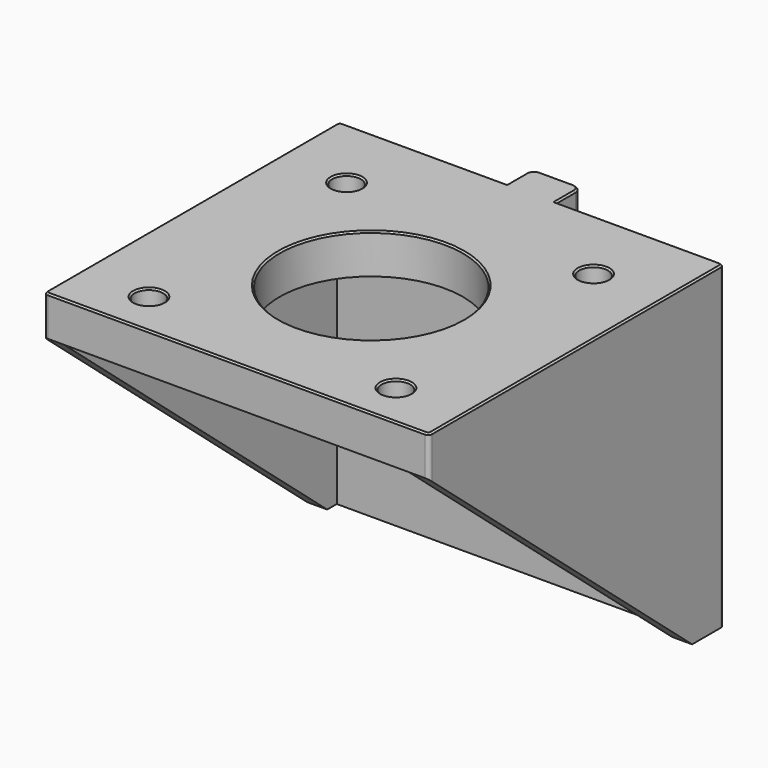
from build123d import *

# Parameters (mm, degrees)
F1_W          = 6.2
F1_H          = 4
F2_DEPTH      = 5
F2_DEPTH_BACK = 35
F3_R          = 1
F5_DEPTH      = 24.151
F5_DEPTH_BACK = 24.151
F6_W          = 43.3
F6_H          = 43.3
F6_R          = 1.8
F6_R_2        = 11.5
F7_DEPTH      = 35.001
F8_DEPTH      = 5.001
F12_R         = 0.5
F13_SIZE      = 0.2


# Not quite as in the source:
# - a feature of the source that left no trace in its solid (it failed there, or was rolled back) is left out


with BuildPart() as f2:
    # F1 (on Top) → F2 (new body, two sides)
    with BuildSketch(Plane.XY) as f2_sk:
        Polygon((-24.15, 25.15), (-24.15, -21.15), (24.15, -21.15), (24.15, 25.15), (3.1, 25.15), (-3.1, 25.15), align=None)
        with Locations((0, 27.15)):
            Rectangle(F1_W, F1_H)
    extrude(amount=F2_DEPTH)
    extrude(f2_sk.sketch, amount=-F2_DEPTH_BACK)

    # F3
    f3_edges = [f2.edges().sort_by_distance(p)[0] for p in [
        (-3.1, 29.15, -15),
        (3.1, 29.15, -15),
    ]]
    fillet(f3_edges, radius=F3_R)

    # F4 (on Right) → F5 (cut, two sides)
    with BuildSketch(Plane.YZ) as f5_sk:
        Polygon((20.15, -35), (-21.15, 0), (-21.15, -35), align=None)
        Polygon((34.9199817246, 9.422104736), (25.15, -7.5), (25.15, -22.5), (34.9199817246, -39.422104736), align=None)
    extrude(amount=-F5_DEPTH, mode=Mode.SUBTRACT)
    extrude(f5_sk.sketch, amount=F5_DEPTH_BACK, mode=Mode.SUBTRACT)

    # F6 (on Top) → F7 (cut, through all)
    with BuildSketch(Plane.XY):
        Rectangle(F6_W, F6_H)
        with Locations((-15.5, -15.5)):
            Circle(F6_R, mode=Mode.SUBTRACT)
        with Locations((15.5, -15.5)):
            Circle(F6_R, mode=Mode.SUBTRACT)
        with Locations((-15.5, 15.5)):
            Circle(F6_R, mode=Mode.SUBTRACT)
        Circle(F6_R_2, mode=Mode.SUBTRACT)
        with Locations((15.5, 15.5)):
            Circle(F6_R, mode=Mode.SUBTRACT)
        with Locations((-15.5, -15.5)):
            Circle(F6_R)
        with Locations((-15.5, 15.5)):
            Circle(F6_R)
        Circle(F6_R_2)
        with Locations((15.5, 15.5)):
            Circle(F6_R)
        with Locations((15.5, -15.5)):
            Circle(F6_R)
    extrude(amount=-F7_DEPTH, mode=Mode.SUBTRACT)

    # F6 (on Top) → F8 (cut, through all)
    with BuildSketch(Plane.XY):
        Circle(F6_R_2)
        with Locations((-15.5, -15.5)):
            Circle(F6_R)
        with Locations((15.5, -15.5)):
            Circle(F6_R)
        with Locations((15.5, 15.5)):
            Circle(F6_R)
        with Locations((-15.5, 15.5)):
            Circle(F6_R)
    extrude(amount=F8_DEPTH, mode=Mode.SUBTRACT)

    # F9 (on Right) → F10 (revolve, cut)
    with BuildSketch(Plane.YZ):
        Polygon((25.15, -17.6), (25.15, -15), (21.65, -15), (21.65, -20.5), (24.55, -17.6), align=None)
    revolve(axis=Axis((0, 23.4, -15), (0, -1, 0)), mode=Mode.SUBTRACT)

    # F12
    f12_edges = [f2.edges().sort_by_distance(p)[0] for p in [
        (24.15, 25.15, -15),
        (-24.15, 25.15, -15),
        (-24.15, -21.15, 2.5),
        (24.15, -21.15, 2.5),
    ]]
    fillet(f12_edges, radius=F12_R)

    # F13
    f13_edges = [f2.edges().sort_by_distance(p)[0] for p in [
        (13.375, 25.15, 5),
        (24.003553, 25.003553, 5),
        (3.1, 26.65, 5),
        (24.15, 2, 5),
        (2.807107, 28.857107, 5),
        (24.003553, -21.003553, 5),
        (0, 29.15, 5),
        (0, -21.15, 5),
        (-2.807107, 28.857107, 5),
        (-24.003553, -21.003553, 5),
        (-3.1, 26.65, 5),
        (-24.15, 2, 5),
        (-13.375, 25.15, 5),
        (-24.003553, 25.003553, 5),
        (-17.3, -15.5, 5),
        (13.7, -15.5, 5),
        (-11.5, 0, 5),
        (-17.3, 15.5, 5),
        (13.7, 15.5, 5),
    ]]
    chamfer(f13_edges, length=F13_SIZE)


solid = f2.part
